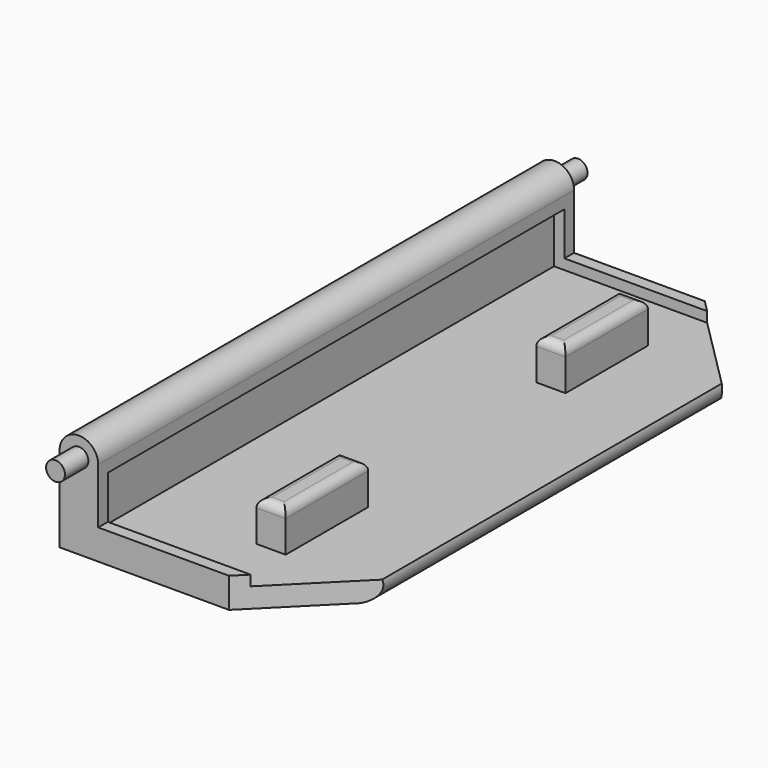
from build123d import *

# Parameters (mm, degrees)
F0_R          = 1.1
F1_DEPTH      = 34.6
F1_DEPTH_BACK = 34.6
F2_DEPTH      = 38
F2_DEPTH_BACK = 38
F4_DEPTH      = 1.2
F5_W          = 3.4
F5_H          = 12
F5_W_2        = 1.2
F5_H_2        = 66.4
F6_DEPTH      = 1.2
F7_DEPTH      = 5
F7_DEPTH_BACK = 5
F8_DEPTH      = 3.5
F9_R          = 1


# Not quite as in the source:
# - a pattern or mirror of a feature is missing from the dataset's text; its kind, count and spacing are read off the source's solid
# - a feature names something its author has since deleted; it is built from what else it names


with BuildPart() as f1:
    # F0 (on Front) → F1 (new body, two sides)
    with BuildSketch(Plane.XZ) as f1_sk:
        with BuildLine():
            ThreePointArc((-12.2672023306, 9.9350791425), (-14.5172023306, 12.1850791425), (-16.7672023306, 9.9350791425))
            Line((-16.7672023306, 9.9350791425), (-16.7672023306, 0))
            Line((-16.7672023306, 0), (10.9618057992, 0))
            ThreePointArc((10.9618057992, 0), (12.9295104862, 1.6360189486), (11.1762294546, 3.5))
            Line((11.1762294546, 3.5), (-12.2672023306, 3.5))
            Line((-12.2672023306, 3.5), (-12.2672023306, 9.9350791425))
        make_face()
        with Locations((-14.5172023306, 9.9350791425)):
            Circle(F0_R, mode=Mode.SUBTRACT)
    extrude(amount=F1_DEPTH)
    extrude(f1_sk.sketch, amount=-F1_DEPTH_BACK)

    # F0 (on Front) → F2 (join, two sides)
    with BuildSketch(Plane.XZ) as f2_sk:
        with Locations((-14.5172023306, 9.9350791425)):
            Circle(F0_R)
    extrude(amount=F2_DEPTH)
    extrude(f2_sk.sketch, amount=-F2_DEPTH_BACK)

    # F3 (on face) → F4 (cut)
    with BuildSketch(Plane.YZ.offset(-12.2672023306)):
        Polygon((-33.2, 4.5), (-33.2, 3.5), (33.2, 3.5), (33.2, 8.5350791425), (-33.2, 8.5350791425), align=None)
    extrude(amount=-F4_DEPTH, mode=Mode.SUBTRACT)

    # F5 (on face) → F6 (cut)
    with BuildSketch(Plane.XY.offset(3.5)):
        Polygon((11.1762294546, 34.6), (2.9438750446, 34.6), (4.3438750446, 33.2), (11.1762294546, 26.36764559), align=None)
        Polygon((4.3438750446, 33.2), (-12.2672023306, 33.2), (-12.2672023306, -33.2), (4.3438750446, -33.2), (11.1762294546, -26.36764559), (11.1762294546, 26.36764559), align=None)
        with Locations((1.2438750446, -20.35)):
            Rectangle(F5_W, F5_H, mode=Mode.SUBTRACT)
        with Locations((1.2438750446, 20.35)):
            Rectangle(F5_W, F5_H, mode=Mode.SUBTRACT)
        with Locations((-12.8672023306, 0)):
            Rectangle(F5_W_2, F5_H_2)
        Polygon((12.9438750446, 24.6), (11.1762294546, 26.36764559), (11.1762294546, -26.36764559), (12.9438750446, -24.6), align=None)
    extrude(amount=-F6_DEPTH, mode=Mode.SUBTRACT)

    # F5 (on face) → F7 (cut, two sides)
    with BuildSketch(Plane.XY.offset(3.5)) as f7_sk:
        Polygon((12.9438750446, 34.6), (11.1762294546, 34.6), (11.1762294546, 26.36764559), (12.9438750446, 24.6), align=None)
        Polygon((12.9438750446, -24.6), (11.1762294546, -26.36764559), (11.1762294546, -34.6), (12.9438750446, -34.6), align=None)
        Polygon((11.1762294546, -26.36764559), (4.3438750446, -33.2), (2.9438750446, -34.6), (11.1762294546, -34.6), align=None)
    f7 = extrude(amount=-F7_DEPTH, mode=Mode.SUBTRACT) + extrude(f7_sk.sketch, amount=F7_DEPTH_BACK, mode=Mode.SUBTRACT)

    # F7_copies: F7 across plane
    add(f7.mirror(Plane.ZX), mode=Mode.SUBTRACT)

    # F5 (on face) → F8 (join)
    with BuildSketch(Plane.XY.offset(3.5)):
        with Locations((1.2438750446, 20.35)):
            Rectangle(F5_W, F5_H)
        with Locations((1.2438750446, -20.35)):
            Rectangle(F5_W, F5_H)
    extrude(amount=F8_DEPTH)

    # F9
    f9_edges = [f1.edges().sort_by_distance(p)[0] for p in [
        (1.243875, -26.35, 7),
        (2.943875, -20.35, 7),
        (1.243875, -14.35, 7),
        (-0.456125, -20.35, 7),
        (-0.456125, 20.35, 7),
        (1.243875, 14.35, 7),
        (2.943875, 20.35, 7),
        (1.243875, 26.35, 7),
    ]]
    fillet(f9_edges, radius=F9_R)


solid = f1.part
